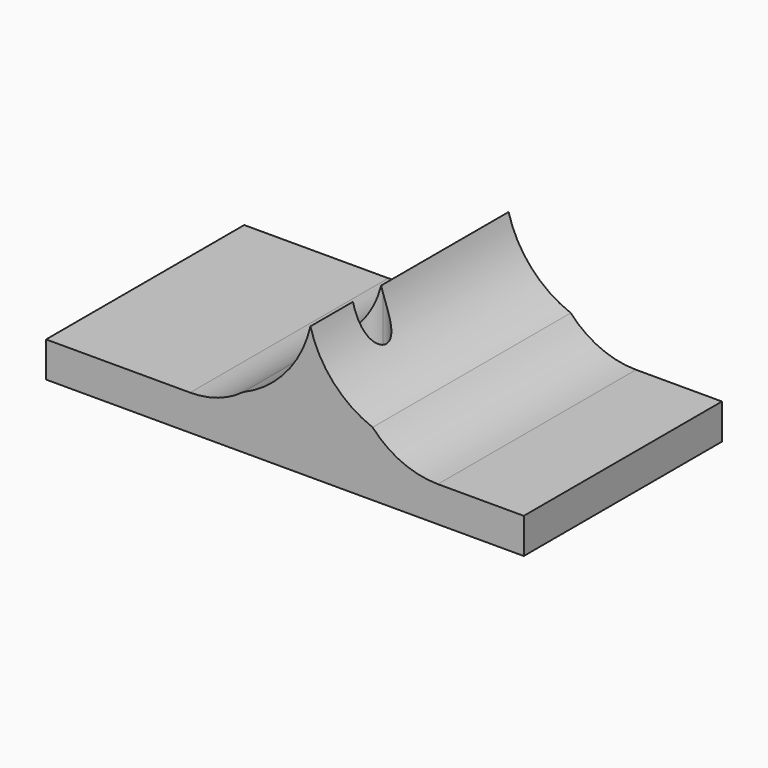
from build123d import *

# Parameters (mm, degrees)
F1_DEPTH    = 14
F4_DEPTH    = 25
F7_DEPTH    = 25
F8_T1_DEPTH = 14
F9_T1_DEPTH = 14


# Not quite as in the source:
# - a fillet or chamfer that OpenCascade refuses, or shapes differently, is made with other operations: its cross-section is extruded or revolved along the edge and cut away or added


with BuildPart() as f1:
    # F0 (on Front) → F1 (new body)
    with BuildSketch(Plane.XZ):
        Polygon((-16.5, 2), (-27, 2), (-27, 0), (0, 0), (0, 2), (-7.5, 2), (-12, 2), align=None)
        Polygon((-12, 9), (-16.5, 2), (-12, 2), align=None)
        Polygon((-12, 9), (-12, 2), (-7.5, 2), align=None)
    extrude(amount=F1_DEPTH)

    # F3 (on face) → F4 (cut)
    with BuildSketch(Plane.XY.offset(9)):
        with BuildLine():
            ThreePointArc((-10.9640486734, -10), (-11.2569418922, -9.2928932188), (-11.9640486734, -9))
            Line((-11.9640486734, -9), (-11.9640486734, -10))
            Line((-11.9640486734, -10), (-11.9640486734, -11))
            ThreePointArc((-11.9640486734, -11), (-11.2569418922, -10.7071067812), (-10.9640486734, -10))
        make_face()
        with BuildLine():
            Line((-11.9640486734, -10), (-11.9640486734, -9))
            ThreePointArc((-11.9640486734, -9), (-12.9640486734, -10), (-11.9640486734, -11))
            Line((-11.9640486734, -11), (-11.9640486734, -10))
        make_face()
    extrude(amount=-F4_DEPTH, mode=Mode.SUBTRACT)

    # F6 (on offset) → F7 (cut)
    with BuildSketch(Plane.XZ.offset(14)):
        with BuildLine():
            Line((-11.884468704, 9.0000648052), (-12.0001798496, 9.0000648052))
            Line((-12.0001798496, 9.0000648052), (-12.253829136, 9.0000648052))
            ThreePointArc((-12.253829136, 9.0000648052), (-12.2044720661, 8.2484912646), (-12.0572486618, 7.5098274869))
            ThreePointArc((-12.0572486618, 7.5098274869), (-11.9278078867, 8.2499547835), (-11.884468704, 9.0000648052))
        make_face()
        with BuildLine():
            Line((-12.253829136, 9.0000648052), (-12.0001798496, 9.0000648052))
            Line((-12.0001798496, 9.0000648052), (-11.884468704, 9.0000648052))
            ThreePointArc((-11.884468704, 9.0000648052), (-11.9278078867, 9.7501748268), (-12.0572486618, 10.4903021234))
            ThreePointArc((-12.0572486618, 10.4903021234), (-12.2044720661, 9.7516383457), (-12.253829136, 9.0000648052))
        make_face()
        with BuildLine():
            ThreePointArc((-12.0572486618, 7.5098274869), (-12.2044720661, 8.2484912646), (-12.253829136, 9.0000648052))
            ThreePointArc((-12.253829136, 9.0000648052), (-12.2044720661, 9.7516383457), (-12.0572486618, 10.4903021234))
            ThreePointArc((-12.0572486618, 10.4903021234), (-24.9106333558, 9.0000648052), (-12.0572486618, 7.5098274869))
        make_face()
        with BuildLine():
            ThreePointArc((-12.0572486618, 10.4903021234), (-11.9278078867, 9.7501748268), (-11.884468704, 9.0000648052))
            ThreePointArc((-11.884468704, 9.0000648052), (-11.9278078867, 8.2499547835), (-12.0572486618, 7.5098274869))
            ThreePointArc((-12.0572486618, 7.5098274869), (-5.7553696033, 3.3025358829), (-0.7600571518, 9.0000648052))
            ThreePointArc((-0.7600571518, 9.0000648052), (-5.7553696033, 14.6975937274), (-12.0572486618, 10.4903021234))
        make_face()
    extrude(amount=-F7_DEPTH, mode=Mode.SUBTRACT)

    # F8: fillet of radius 5 on 1 edges, made by hand

    # F8_s2 → F8_t1 (join)
    with BuildSketch(Plane.XZ):
        with BuildLine():
            ThreePointArc((-18.8598420152, 2), (-17.2756076516, 2.2576164768), (-15.854623238, 3.0039194075))
            Line((-15.854623238, 3.0039194075), (-16.5, 2))
            Line((-16.5, 2), (-18.8598420152, 2))
        make_face()
    extrude(amount=F8_T1_DEPTH)

    # F9: fillet of radius 5 on 1 edges, made by hand

    # F9_s2 → F9_t1 (join)
    with BuildSketch(Plane.XZ):
        with BuildLine():
            ThreePointArc((-8.5459751266, 3.6270724192), (-6.8718408683, 2.4248148724), (-4.8549915809, 2))
            Line((-4.8549915809, 2), (-7.5, 2))
            Line((-7.5, 2), (-8.5459751266, 3.6270724192))
        make_face()
    extrude(amount=F9_T1_DEPTH)


solid = f1.part
